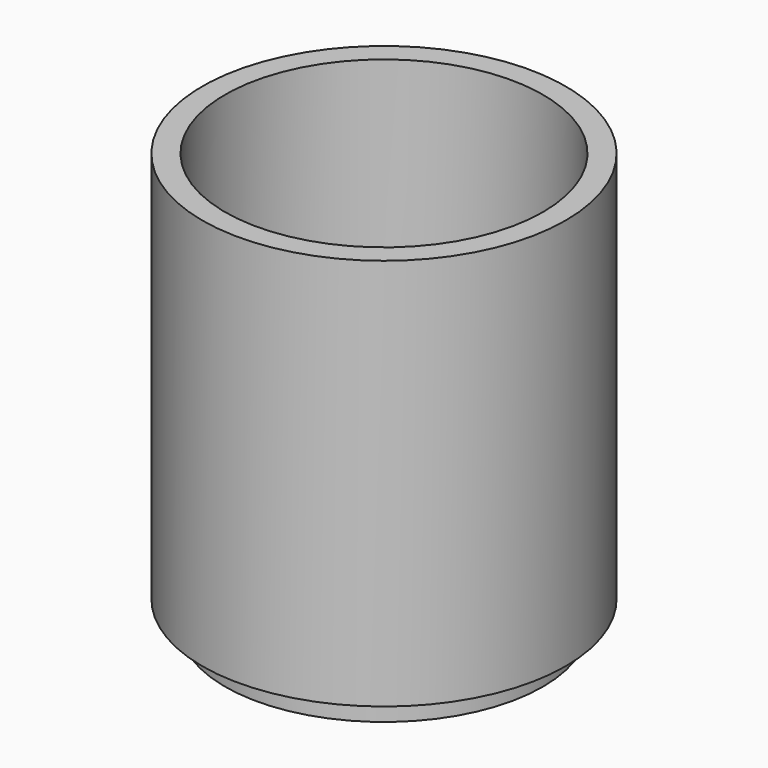
from build123d import *

# Parameters (mm, degrees)
F0_R     = 50.8
F0_R_2   = 44.45
F1_DEPTH = 54.864
F3_DEPTH = 61.976


# Not quite as in the source:
# - the program builds the solid bodies; features that only make, move or delete a surface that nothing else refers to are left out


with BuildPart() as f1:
    # F0 (on Top) → F1 (new body, symmetric)
    with BuildSketch(Plane.XY):
        Circle(F0_R)
        Circle(F0_R_2, mode=Mode.SUBTRACT)
    extrude(amount=F1_DEPTH, both=True)

    # F0 (on Top) → F3 (join)
    with BuildSketch(Plane.XY):
        Circle(F0_R_2)
    extrude(amount=-F3_DEPTH)


solid = f1.part
